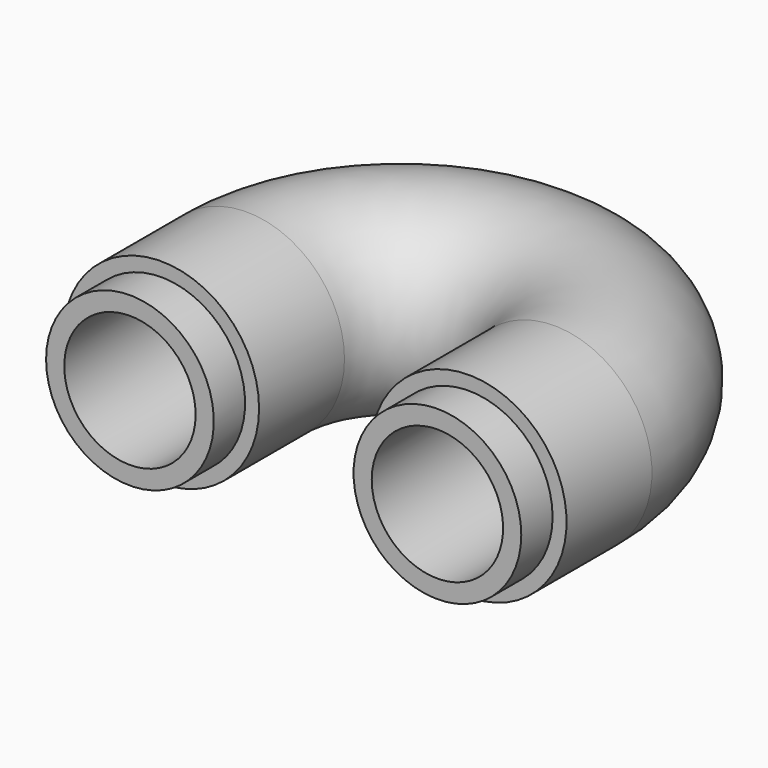
from build123d import *

# Parameters (mm, degrees)
F1_R     = 8.89
F1_R_2   = 5.969
F3_DEPTH = 3.556
F5_R     = 8.89
F5_R_2   = 7.62
F7_DEPTH = 3.556


# Not quite as in the source:
# - a feature of the source that left no trace in its solid (it failed there, or was rolled back) is left out
# - a pattern or mirror of a feature is missing from the dataset's text; its kind, count and spacing are read off the source's solid


with BuildPart() as f2:
    # F2: sweep along a path in F0
    with BuildLine(Plane.XY) as f2_path:
        Line((0, 0), (0, 9.7015046))
        ThreePointArc((0, 9.7015046), (13.97, 23.6715046), (27.94, 9.7015046))
        Line((27.94, 9.7015046), (27.94, 0))
        Line((27.94, 0), (27.94, -3.556))
    # F1 (on Front) → F2 (sweep)
    with BuildSketch(Plane.XZ):
        Circle(F1_R)
        Circle(F1_R_2, mode=Mode.SUBTRACT)
    sweep(path=f2_path.line)

    # F3 (add): a face of the model
    f3_faces = [f2.faces().sort_by_distance(p)[0] for p in [
        (-8.6385528286, 0, 0),
    ]]
    extrude(f3_faces, amount=F3_DEPTH)

    # F5 (on face) → F7 (cut)
    with BuildSketch(Plane.XZ.offset(3.556)):
        with Locations((27.94, 0)):
            Circle(F5_R)
        with Locations((27.94, 0)):
            Circle(F5_R_2, mode=Mode.SUBTRACT)
    f7 = extrude(amount=-F7_DEPTH, mode=Mode.SUBTRACT)

    # F7_copies: F7 across plane
    add(f7.mirror(Plane(origin=(13.97, 0, 0), x_dir=(0, 0, -1), z_dir=(-1, 0, 0))), mode=Mode.SUBTRACT)


solid = f2.part
